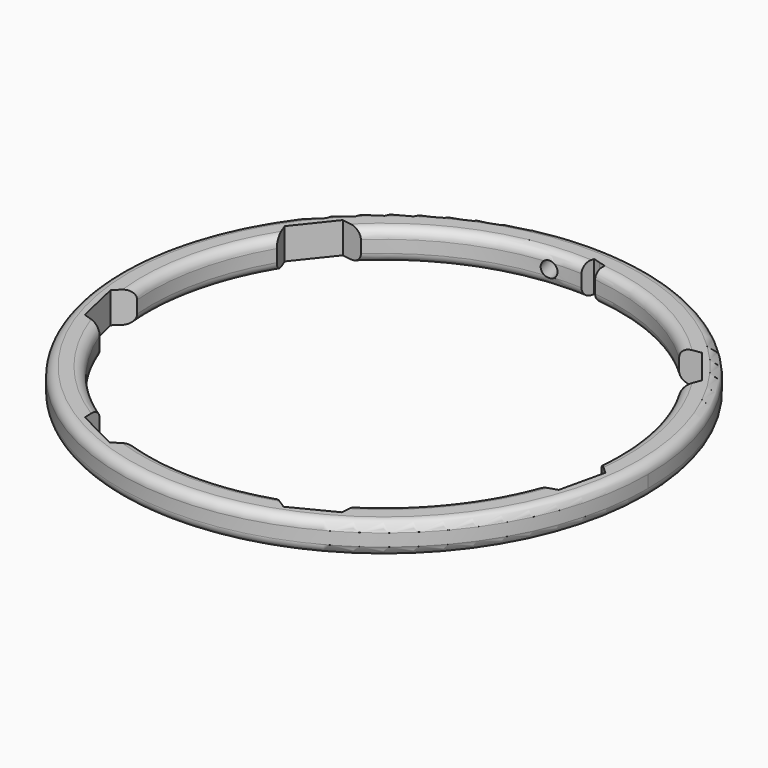
from build123d import *

# Parameters (mm, degrees)
F0_R          = 85
F1_DEPTH      = 10
F3_R          = 2.5
F4_DEPTH      = 5.1820354925
F4_DEPTH_BACK = 5.8422830271
F7_DEPTH      = 10
F8_T2_ANGLE   = 57.3924416143
F8_T4_ANGLE   = 46.2655120584
F8_T6_ANGLE   = 46.4941868537
F8_T8_ANGLE   = 45.7826972377
F8_T10_ANGLE  = 46.4941868537
F8_T12_ANGLE  = 46.2655120584
F8_T16_ANGLE  = 48.1827650259
F8_T20_ANGLE  = 46.4941868537
F8_T22_ANGLE  = 45.7826972377
F8_T24_ANGLE  = 46.4941868537
F8_T26_ANGLE  = 46.2655120584
F8_T28_ANGLE  = 48.1827650259
F8_T30_ANGLE  = 57.3924416143
F8_T32_ANGLE  = 46.2655120584


# Not quite as in the source:
# - a fillet or chamfer that OpenCascade refuses, or shapes differently, is made with other operations: its cross-section is extruded or revolved along the edge and cut away or added


with BuildPart() as f1:
    # F0 (on Top) → F1 (new body)
    with BuildSketch(Plane.XY):
        Circle(F0_R)
        with BuildLine():
            ThreePointArc((64.7810828293, 37.7943290384), (72.4002113678, 19.5757348241), (75, 0))
            ThreePointArc((75, 0), (74.9409977062, -2.9743676293), (74.7640836588, -5.9440554048))
            Line((74.7640836588, -5.9440554048), (79.6631399792, -10.4897153751))
            Line((79.6631399792, -10.4897153751), (76.3253259699, -25.1136340579))
            Line((76.3253259699, -25.1136340579), (69.9391407984, -27.0835113007))
            ThreePointArc((69.9391407984, -27.0835113007), (58.5439321667, -46.8786519267), (41.7189859151, -62.325967415))
            Line((41.7189859151, -62.325967415), (41.3909329339, -68.6680408053))
            Line((41.3909329339, -68.6680408053), (28.0304653249, -75.4869780591))
            Line((28.0304653249, -75.4869780591), (22.1298761331, -71.6607883178))
            ThreePointArc((22.1298761331, -71.6607883178), (0, -75), (-22.1298761331, -71.6607883178))
            Line((-22.1298761331, -71.6607883178), (-28.0304653249, -75.4869780591))
            Line((-28.0304653249, -75.4869780591), (-41.3909329339, -68.6680408053))
            Line((-41.3909329339, -68.6680408053), (-41.7189859151, -62.325967415))
            ThreePointArc((-41.7189859151, -62.325967415), (-58.5439321667, -46.8786519267), (-69.9391407984, -27.0835113007))
            Line((-69.9391407984, -27.0835113007), (-76.3253259699, -25.1136340579))
            Line((-76.3253259699, -25.1136340579), (-79.6631399792, -10.4897153751))
            Line((-79.6631399792, -10.4897153751), (-74.7640836588, -5.9440554048))
            ThreePointArc((-74.7640836588, -5.9440554048), (-73.1195934136, 16.6890700467), (-64.7810828293, 37.7943290384))
            Line((-64.7810828293, 37.7943290384), (-67.2226921114, 44.0154480302))
            Line((-67.2226921114, 44.0154480302), (-57.8703450835, 55.7429202672))
            Line((-57.8703450835, 55.7429202672), (-51.2618933556, 54.7468564357))
            ThreePointArc((-51.2618933556, 54.7468564357), (0, 75), (51.2618933556, 54.7468564357))
            Line((51.2618933556, 54.7468564357), (57.8703450835, 55.7429202672))
            Line((57.8703450835, 55.7429202672), (67.2226921114, 44.0154480302))
            Line((67.2226921114, 44.0154480302), (64.7810828293, 37.7943290384))
        make_face(mode=Mode.SUBTRACT)
    extrude(amount=F1_DEPTH)

    # F3 (on line) → F4 (cut, two sides)
    with BuildSketch(Plane(origin=(-21.1440301916, 76.2096754052, 0), x_dir=(0.9636004367, 0.2673465885, 0), z_dir=(0.2673465885, -0.9636004367, 0))) as f4_sk:
        with Locations((13.6198922992, 5)):
            Circle(F3_R)
    extrude(amount=-F4_DEPTH, mode=Mode.SUBTRACT)
    extrude(f4_sk.sketch, amount=F4_DEPTH_BACK, mode=Mode.SUBTRACT)

    # F6 (on face) → F7 (cut, through all)
    with BuildSketch(Plane.XY.offset(10)):
        with BuildLine():
            Line((9.1547645904, 77.4242299714), (6.9384835859, 78.0391271248))
            Line((6.9384835859, 78.0391271248), (6.0279733518, 74.757364435))
            ThreePointArc((6.0279733518, 74.757364435), (7.1912208158, 74.6544462385), (8.352724825, 74.5334286612))
            Line((8.352724825, 74.5334286612), (9.1547645904, 77.4242299714))
        make_face()
        with BuildLine():
            Line((6.9384835859, 78.0391271248), (4.7222025815, 78.6540242783))
            Line((4.7222025815, 78.6540242783), (3.6833014209, 74.9095006701))
            ThreePointArc((3.6833014209, 74.9095006701), (4.8562331891, 74.8426148609), (6.0279733518, 74.757364435))
            Line((6.0279733518, 74.757364435), (6.9384835859, 78.0391271248))
        make_face()
    extrude(amount=-F7_DEPTH, mode=Mode.SUBTRACT)

    # F8: fillet of radius 3 on 16 edges, made by hand

    # F8_s1 → F8_t2 (revolve, cut)
    with BuildSketch(Plane(origin=(0, 0, 0), x_dir=(0, 0, 1), z_dir=(-0.6580681265, -0.7529583925, 0))):
        with BuildLine():
            ThreePointArc((10, 78), (9.1213203436, 75.8786796564), (7, 75))
            Line((7, 75), (10, 75))
            Line((10, 75), (10, 78))
        make_face()
    revolve(axis=Axis((0, 0, 10), (0, 0, -1)), revolution_arc=F8_T2_ANGLE, mode=Mode.SUBTRACT)

    # F8_s3 → F8_t4 (revolve, cut)
    with BuildSketch(Plane(origin=(0, 0, 0), x_dir=(0, 0, 1), z_dir=(-0.1783834275, -0.9839610525, 0))):
        with BuildLine():
            ThreePointArc((10, -78), (9.1213203436, -75.8786796564), (7, -75))
            Line((7, -75), (10, -75))
            Line((10, -75), (10, -78))
        make_face()
    revolve(axis=Axis((0, 0, 10), (0, 0, 1)), revolution_arc=F8_T4_ANGLE, mode=Mode.SUBTRACT)

    # F8_s5 → F8_t6 (revolve, cut)
    with BuildSketch(Plane(origin=(0, 0, 0), x_dir=(0, 0, 1), z_dir=(0.2662067095, 0.9639159651, 0))):
        with BuildLine():
            ThreePointArc((10, 78), (9.1213203436, 75.8786796564), (7, 75))
            Line((7, 75), (10, 75))
            Line((10, 75), (10, 78))
        make_face()
    revolve(axis=Axis((0, 0, 10), (0, 0, -1)), revolution_arc=F8_T6_ANGLE, mode=Mode.SUBTRACT)

    # F8_s7 → F8_t8 (revolve, cut)
    with BuildSketch(Plane(origin=(0, 0, 0), x_dir=(0, 0, 1), z_dir=(0.9212441509, 0.3889848512, 0))):
        with BuildLine():
            ThreePointArc((10, 78), (9.1213203436, 75.8786796564), (7, 75))
            Line((7, 75), (10, 75))
            Line((10, 75), (10, 78))
        make_face()
    revolve(axis=Axis((0, 0, 10), (0, 0, -1)), revolution_arc=F8_T8_ANGLE, mode=Mode.SUBTRACT)

    # F8_s9 → F8_t10 (revolve, cut)
    with BuildSketch(Plane(origin=(0, 0, 0), x_dir=(0, 0, 1), z_dir=(0.8823968112, -0.4705059698, 0))):
        with BuildLine():
            ThreePointArc((10, 78), (9.1213203436, 75.8786796564), (7, 75))
            Line((7, 75), (10, 75))
            Line((10, 75), (10, 78))
        make_face()
    revolve(axis=Axis((0, 0, 10), (0, 0, -1)), revolution_arc=F8_T10_ANGLE, mode=Mode.SUBTRACT)

    # F8_s11 → F8_t12 (revolve, cut)
    with BuildSketch(Plane(origin=(0, 0, 0), x_dir=(0, 0, 1), z_dir=(0.1783834275, -0.9839610525, 0))):
        with BuildLine():
            ThreePointArc((10, 78), (9.1213203436, 75.8786796564), (7, 75))
            Line((7, 75), (10, 75))
            Line((10, 75), (10, 78))
        make_face()
    revolve(axis=Axis((0, 0, 10), (0, 0, -1)), revolution_arc=F8_T12_ANGLE, mode=Mode.SUBTRACT)

    # F8_s13 → F8_t14 (revolve, cut)
    with BuildSketch(Plane.XZ):
        with BuildLine():
            ThreePointArc((85, 7), (84.1213203436, 9.1213203436), (82, 10))
            Line((82, 10), (85, 10))
            Line((85, 10), (85, 7))
        make_face()
    revolve(axis=Axis((0, 0, 10), (0, 0, 1)), mode=Mode.SUBTRACT)

    # F8_s15 → F8_t16 (revolve, cut)
    with BuildSketch(Plane(origin=(0, 0, 0), x_dir=(0, 0, 1), z_dir=(-0.9999327846, 0.011594236, 0))):
        with BuildLine():
            ThreePointArc((10, 78), (9.1213203436, 75.8786796564), (7, 75))
            Line((7, 75), (10, 75))
            Line((10, 75), (10, 78))
        make_face()
    revolve(axis=Axis((0, 0, 10), (0, 0, -1)), revolution_arc=F8_T16_ANGLE, mode=Mode.SUBTRACT)

    # F8_s17 → F8_t18 (revolve, cut)
    with BuildSketch(Plane.XZ):
        with BuildLine():
            ThreePointArc((85, 3), (84.1213203436, 0.8786796564), (82, 0))
            Line((82, 0), (85, 0))
            Line((85, 0), (85, 3))
        make_face()
    revolve(axis=Axis((0, 0, 0), (0, 0, 1)), mode=Mode.SUBTRACT)

    # F8_s19 → F8_t20 (revolve, cut)
    with BuildSketch(Plane(origin=(0, 0, 0), x_dir=(0, 0, 1), z_dir=(0.8823968112, -0.4705059698, 0))):
        with BuildLine():
            ThreePointArc((0, 78), (0.8786796564, 75.8786796564), (3, 75))
            Line((3, 75), (0, 75))
            Line((0, 75), (0, 78))
        make_face()
    revolve(axis=Axis((0, 0, 0), (0, 0, -1)), revolution_arc=F8_T20_ANGLE, mode=Mode.SUBTRACT)

    # F8_s21 → F8_t22 (revolve, cut)
    with BuildSketch(Plane(origin=(0, 0, 0), x_dir=(0, 0, 1), z_dir=(0.9212441509, 0.3889848512, 0))):
        with BuildLine():
            ThreePointArc((0, 78), (0.8786796564, 75.8786796564), (3, 75))
            Line((3, 75), (0, 75))
            Line((0, 75), (0, 78))
        make_face()
    revolve(axis=Axis((0, 0, 0), (0, 0, -1)), revolution_arc=F8_T22_ANGLE, mode=Mode.SUBTRACT)

    # F8_s23 → F8_t24 (revolve, cut)
    with BuildSketch(Plane(origin=(0, 0, 0), x_dir=(0, 0, 1), z_dir=(0.2662067095, 0.9639159651, 0))):
        with BuildLine():
            ThreePointArc((0, 78), (0.8786796564, 75.8786796564), (3, 75))
            Line((3, 75), (0, 75))
            Line((0, 75), (0, 78))
        make_face()
    revolve(axis=Axis((0, 0, 0), (0, 0, -1)), revolution_arc=F8_T24_ANGLE, mode=Mode.SUBTRACT)

    # F8_s25 → F8_t26 (revolve, cut)
    with BuildSketch(Plane(origin=(0, 0, 0), x_dir=(0, 0, 1), z_dir=(-0.5876426153, 0.809120607, 0))):
        with BuildLine():
            ThreePointArc((0, 78), (0.8786796564, 75.8786796564), (3, 75))
            Line((3, 75), (0, 75))
            Line((0, 75), (0, 78))
        make_face()
    revolve(axis=Axis((0, 0, 0), (0, 0, -1)), revolution_arc=F8_T26_ANGLE, mode=Mode.SUBTRACT)

    # F8_s27 → F8_t28 (revolve, cut)
    with BuildSketch(Plane(origin=(0, 0, 0), x_dir=(0, 0, 1), z_dir=(-0.9999327846, 0.011594236, 0))):
        with BuildLine():
            ThreePointArc((0, 78), (0.8786796564, 75.8786796564), (3, 75))
            Line((3, 75), (0, 75))
            Line((0, 75), (0, 78))
        make_face()
    revolve(axis=Axis((0, 0, 0), (0, 0, -1)), revolution_arc=F8_T28_ANGLE, mode=Mode.SUBTRACT)

    # F8_s29 → F8_t30 (revolve, cut)
    with BuildSketch(Plane(origin=(0, 0, 0), x_dir=(0, 0, 1), z_dir=(-0.6580681265, -0.7529583925, 0))):
        with BuildLine():
            ThreePointArc((0, 78), (0.8786796564, 75.8786796564), (3, 75))
            Line((3, 75), (0, 75))
            Line((0, 75), (0, 78))
        make_face()
    revolve(axis=Axis((0, 0, 0), (0, 0, -1)), revolution_arc=F8_T30_ANGLE, mode=Mode.SUBTRACT)

    # F8_s31 → F8_t32 (revolve, cut)
    with BuildSketch(Plane(origin=(0, 0, 0), x_dir=(0, 0, 1), z_dir=(0.1783834275, -0.9839610525, 0))):
        with BuildLine():
            ThreePointArc((0, 78), (0.8786796564, 75.8786796564), (3, 75))
            Line((3, 75), (0, 75))
            Line((0, 75), (0, 78))
        make_face()
    revolve(axis=Axis((0, 0, 0), (0, 0, -1)), revolution_arc=F8_T32_ANGLE, mode=Mode.SUBTRACT)


solid = f1.part
